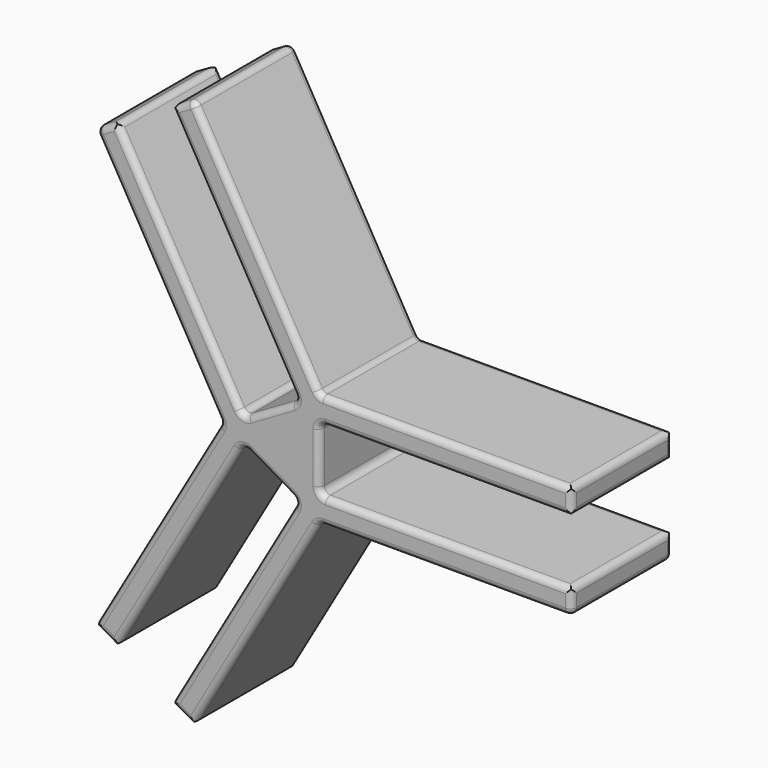
from build123d import *

# Parameters (mm, degrees)
F1_DEPTH    = 12.7
F2_R        = 0.635
F3_T1_DEPTH = 14.605


# Not quite as in the source:
# - a fillet or chamfer that OpenCascade refuses, or shapes differently, is made with other operations: its cross-section is extruded or revolved along the edge and cut away or added


with BuildPart() as f1:
    # F0 (on Front) → F1 (new body)
    with BuildSketch(Plane.XZ):
        with BuildLine():
            Line((3.9345567884, 3.175), (28.6995567884, 3.175))
            Line((28.6995567884, 3.175), (28.6995567884, 5.715))
            Line((28.6995567884, 5.715), (3.2995567884, 5.715))
            Line((3.2995567884, 5.715), (-9.4004432116, 27.7120452561))
            Line((-9.4004432116, 27.7120452561), (-11.6001477372, 26.4420452561))
            Line((-11.6001477372, 26.4420452561), (0.7823522628, 4.9949261314))
            ThreePointArc((0.7823522628, 4.9949261314), (0.8457890311, 4.5130760378), (0.5499261314, 4.1275))
            Line((0.5499261314, 4.1275), (-3.8494829198, 1.5875))
            ThreePointArc((-3.8494829198, 1.5875), (-4.3313330135, 1.5240632317), (-4.7169090512, 1.8199261314))
            Line((-4.7169090512, 1.8199261314), (-17.0994090512, 23.2670452561))
            Line((-17.0994090512, 23.2670452561), (-19.2991135768, 21.9970452561))
            Line((-19.2991135768, 21.9970452561), (-6.5991135768, 0))
            Line((-6.5991135768, 0), (-19.2991135768, -21.9970452561))
            Line((-19.2991135768, -21.9970452561), (-17.0994090512, -23.2670452561))
            Line((-17.0994090512, -23.2670452561), (-4.7169090512, -1.8199261314))
            ThreePointArc((-4.7169090512, -1.8199261314), (-4.3313330135, -1.5240632317), (-3.8494829198, -1.5875))
            Line((-3.8494829198, -1.5875), (0.5499261314, -4.1275))
            ThreePointArc((0.5499261314, -4.1275), (0.8457890311, -4.5130760378), (0.7823522628, -4.9949261314))
            Line((0.7823522628, -4.9949261314), (-11.6001477372, -26.4420452561))
            Line((-11.6001477372, -26.4420452561), (-9.4004432116, -27.7120452561))
            Line((-9.4004432116, -27.7120452561), (3.2995567884, -5.715))
            Line((3.2995567884, -5.715), (28.6995567884, -5.715))
            Line((28.6995567884, -5.715), (28.6995567884, -3.175))
            Line((28.6995567884, -3.175), (3.9345567884, -3.175))
            ThreePointArc((3.9345567884, -3.175), (3.4855439824, -2.9890128061), (3.2995567884, -2.54))
            Line((3.2995567884, -2.54), (3.2995567884, 2.54))
            ThreePointArc((3.2995567884, 2.54), (3.4855439824, 2.9890128061), (3.9345567884, 3.175))
        make_face()
    extrude(amount=F1_DEPTH)

    # F2
    f2_edges = [f1.edges().sort_by_distance(p)[0] for p in [
        (3.299557, -6.35, 5.715),
        (-9.400443, -6.35, 27.712045),
        (-3.050443, 0, 16.713523),
        (-3.050443, -12.7, 16.713523),
        (28.699557, -12.7, -4.445),
        (16.317057, -12.7, -3.175),
        (3.485544, -12.7, -2.989013),
        (3.299557, -12.7, 0),
        (3.485544, -12.7, 2.989013),
        (16.317057, -12.7, 3.175),
        (28.699557, -12.7, 4.445),
        (15.999557, -12.7, 5.715),
        (-10.500295, -12.7, 27.077045),
        (-5.408898, -12.7, 15.718486),
        (0.845789, -12.7, 4.513076),
        (-1.649778, -12.7, 2.8575),
        (-4.331333, -12.7, 1.524063),
        (-10.908159, -12.7, 12.543486),
        (-18.199261, -12.7, 22.632045),
        (-12.949114, -12.7, 10.998523),
        (-12.949114, -12.7, -10.998523),
        (-18.199261, -12.7, -22.632045),
        (-10.908159, -12.7, -12.543486),
        (-4.331333, -12.7, -1.524063),
        (-1.649778, -12.7, -2.8575),
        (0.845789, -12.7, -4.513076),
        (-5.408898, -12.7, -15.718486),
        (-10.500295, -12.7, -27.077045),
        (-3.050443, -12.7, -16.713523),
        (15.999557, -12.7, -5.715),
        (28.699557, 0, -4.445),
        (16.317057, 0, -3.175),
        (3.485544, 0, -2.989013),
        (3.299557, 0, 0),
        (3.485544, 0, 2.989013),
        (16.317057, 0, 3.175),
        (28.699557, 0, 4.445),
        (15.999557, 0, 5.715),
        (-10.500295, 0, 27.077045),
        (-5.408898, 0, 15.718486),
        (0.845789, 0, 4.513076),
        (-1.649778, 0, 2.8575),
        (-4.331333, 0, 1.524063),
        (-10.908159, 0, 12.543486),
        (-18.199261, 0, 22.632045),
        (-12.949114, 0, 10.998523),
        (-12.949114, 0, -10.998523),
        (-18.199261, 0, -22.632045),
        (-10.908159, 0, -12.543486),
        (-4.331333, 0, -1.524063),
        (-1.649778, 0, -2.8575),
        (0.845789, 0, -4.513076),
        (-5.408898, 0, -15.718486),
        (-10.500295, 0, -27.077045),
        (-3.050443, 0, -16.713523),
        (15.999557, 0, -5.715),
        (-19.299114, -6.35, 21.997045),
        (-6.599114, -6.35, 0),
        (3.299557, -6.35, -5.715),
        (28.699557, -6.35, -5.715),
    ]]
    fillet(f2_edges, radius=F2_R)

    # F3: fillet of radius 0.635 on 24 edges, made by hand

    # F3_s2 → F3_t1 (cut)
    with BuildSketch(Plane.XZ.offset(-0.9525)):
        with BuildLine():
            ThreePointArc((28.6995567884, -3.81), (28.5135695945, -3.3609871939), (28.0645567884, -3.175))
            Line((28.0645567884, -3.175), (28.6995567884, -3.175))
            Line((28.6995567884, -3.175), (28.6995567884, -3.81))
        make_face()
        with BuildLine():
            ThreePointArc((28.6995567884, 3.81), (28.5135695945, 3.3609871939), (28.0645567884, 3.175))
            Line((28.0645567884, 3.175), (28.6995567884, 3.175))
            Line((28.6995567884, 3.175), (28.6995567884, 3.81))
        make_face()
        with BuildLine():
            ThreePointArc((28.0645567884, 5.715), (28.5135695945, 5.5290128061), (28.6995567884, 5.08))
            Line((28.6995567884, 5.08), (28.6995567884, 5.715))
            Line((28.6995567884, 5.715), (28.0645567884, 5.715))
        make_face()
        with BuildLine():
            ThreePointArc((-11.0502216058, -26.7595452561), (-11.3460845055, -26.3739692184), (-11.2826477372, -25.8921191247))
            Line((-11.2826477372, -25.8921191247), (-11.6001477372, -26.4420452561))
            Line((-11.6001477372, -26.4420452561), (-11.0502216058, -26.7595452561))
        make_face()
        with BuildLine():
            ThreePointArc((-9.0829432116, -27.1621191247), (-9.4685192493, -27.4579820244), (-9.950369343, -27.3945452561))
            Line((-9.950369343, -27.3945452561), (-9.4004432116, -27.7120452561))
            Line((-9.4004432116, -27.7120452561), (-9.0829432116, -27.1621191247))
        make_face()
        with BuildLine():
            ThreePointArc((-18.9816135768, -21.4471191247), (-19.0450503451, -21.9289692184), (-18.7491874454, -22.3145452561))
            Line((-18.7491874454, -22.3145452561), (-19.2991135768, -21.9970452561))
            Line((-19.2991135768, -21.9970452561), (-18.9816135768, -21.4471191247))
        make_face()
        with BuildLine():
            ThreePointArc((-17.6493351826, -22.9495452561), (-17.167485089, -23.0129820244), (-16.7819090512, -22.7171191247))
            Line((-16.7819090512, -22.7171191247), (-17.0994090512, -23.2670452561))
            Line((-17.0994090512, -23.2670452561), (-17.6493351826, -22.9495452561))
        make_face()
        with BuildLine():
            ThreePointArc((-11.0502216058, 26.7595452561), (-11.3460845055, 26.3739692184), (-11.2826477372, 25.8921191247))
            Line((-11.2826477372, 25.8921191247), (-11.6001477372, 26.4420452561))
            Line((-11.6001477372, 26.4420452561), (-11.0502216058, 26.7595452561))
        make_face()
        with BuildLine():
            ThreePointArc((-16.7819090512, 22.7171191247), (-17.167485089, 23.0129820244), (-17.6493351826, 22.9495452561))
            Line((-17.6493351826, 22.9495452561), (-17.0994090512, 23.2670452561))
            Line((-17.0994090512, 23.2670452561), (-16.7819090512, 22.7171191247))
        make_face()
    extrude(amount=F3_T1_DEPTH, mode=Mode.SUBTRACT)


solid = f1.part
